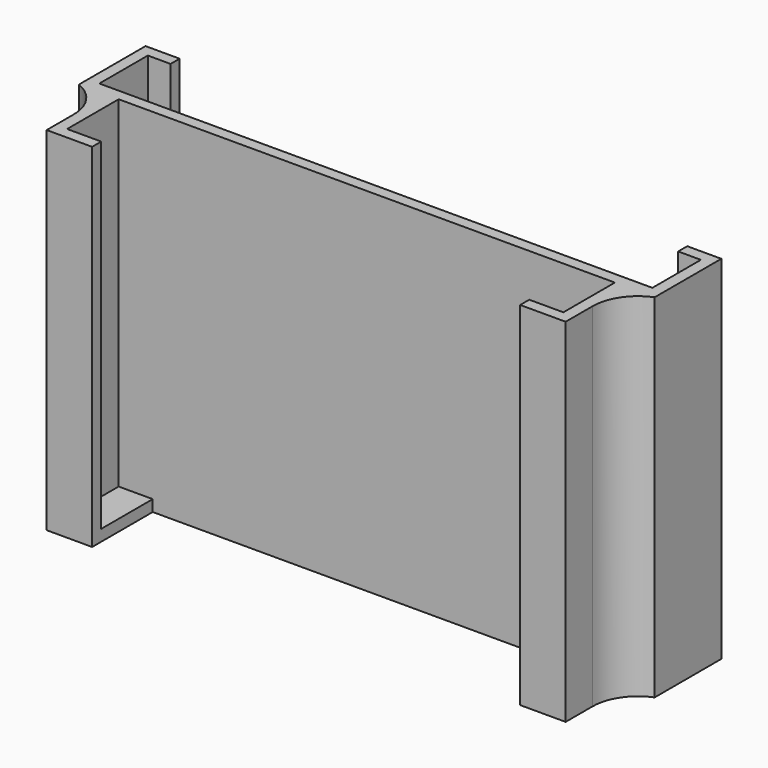
from build123d import *

# Parameters (mm, degrees)
F1_DEPTH    = 45
F2_T1_DEPTH = 45
F3_W        = 4.5
F3_H        = 8.5
F4_DEPTH    = 1.5


# Not quite as in the source:
# - a fillet or chamfer that OpenCascade refuses, or shapes differently, is made with other operations: its cross-section is extruded or revolved along the edge and cut away or added


with BuildPart() as f1:
    # F0 (on Top) → F1 (new body)
    with BuildSketch(Plane.XY):
        Polygon((36.5, 0), (0, 0), (-36.5, 0), (-36.5, 8), (-33.5, 8), (-33.5, 9.5), (-38, 9.5), (-38, -1.5), (-34.25, -1.5), (-32.75, -1.5), (0, -1.5), (32.75, -1.5), (34.25, -1.5), (38, -1.5), (38, 9.5), (33.5, 9.5), (33.5, 8), (36.5, 8), align=None)
        Polygon((-32.75, -1.5), (-34.25, -1.5), (-34.25, -11.5), (-28.25, -11.5), (-28.25, -10), (-32.75, -10), align=None)
        Polygon((34.25, -11.5), (34.25, -1.5), (32.75, -1.5), (32.75, -10), (28.25, -10), (28.25, -11.5), align=None)
    extrude(amount=F1_DEPTH)

    # F2: fillet of radius 6 on 2 edges, made by hand

    # F2_s2 → F2_t1 (join)
    with BuildSketch(Plane.XY):
        with BuildLine():
            ThreePointArc((-38, -1.5), (-35.2750628145, -3.7080468991), (-34.25, -7.0621488653))
            Line((-34.25, -7.0621488653), (-34.25, -1.5))
            Line((-34.25, -1.5), (-38, -1.5))
        make_face()
        with BuildLine():
            ThreePointArc((34.25, -7.0621488653), (35.2750628145, -3.7080468991), (38, -1.5))
            Line((38, -1.5), (34.25, -1.5))
            Line((34.25, -1.5), (34.25, -7.0621488653))
        make_face()
    extrude(amount=F2_T1_DEPTH)

    # F3 (on face) → F4 (join)
    with BuildSketch(Plane(origin=(0, 0, 0), x_dir=(1, 0, 0), z_dir=(0, 0, -1))):
        with BuildLine():
            Line((-38, -9.5), (-33.5, -9.5))
            Line((-33.5, -9.5), (-33.5, -8))
            Line((-33.5, -8), (-36.5, -8))
            Line((-36.5, -8), (-36.5, 0))
            Line((-36.5, 0), (-20, 0))
            Line((-20, 0), (20, 0))
            Line((20, 0), (36.5, 0))
            Line((36.5, 0), (36.5, -8))
            Line((36.5, -8), (33.5, -8))
            Line((33.5, -8), (33.5, -9.5))
            Line((33.5, -9.5), (38, -9.5))
            Line((38, -9.5), (38, 1.5))
            ThreePointArc((38, 1.5), (35.2750628145, 3.7080468991), (34.25, 7.0621488653))
            Line((34.25, 7.0621488653), (34.25, 11.5))
            Line((34.25, 11.5), (28.25, 11.5))
            Line((28.25, 11.5), (28.25, 10))
            Line((28.25, 10), (32.75, 10))
            Line((32.75, 10), (32.75, 1.5))
            Line((32.75, 1.5), (28.25, 1.5))
            Line((28.25, 1.5), (-28.25, 1.5))
            Line((-28.25, 1.5), (-32.75, 1.5))
            Line((-32.75, 1.5), (-32.75, 10))
            Line((-32.75, 10), (-28.25, 10))
            Line((-28.25, 10), (-28.25, 11.5))
            Line((-28.25, 11.5), (-34.25, 11.5))
            Line((-34.25, 11.5), (-34.25, 7.0621488653))
            ThreePointArc((-34.25, 7.0621488653), (-35.2750628145, 3.7080468991), (-38, 1.5))
            Line((-38, 1.5), (-38, -9.5))
        make_face()
        with Locations((-30.5, 5.75)):
            Rectangle(F3_W, F3_H)
        Polygon((-33.5, -8), (-33.5, -9.5), (-20, -9.5), (-20, 0), (-36.5, 0), (-36.5, -8), align=None)
        Polygon((36.5, 0), (20, 0), (20, -9.5), (33.5, -9.5), (33.5, -8), (36.5, -8), align=None)
        with Locations((30.5, 5.75)):
            Rectangle(F3_W, F3_H)
    extrude(amount=F4_DEPTH)


solid = f1.part
